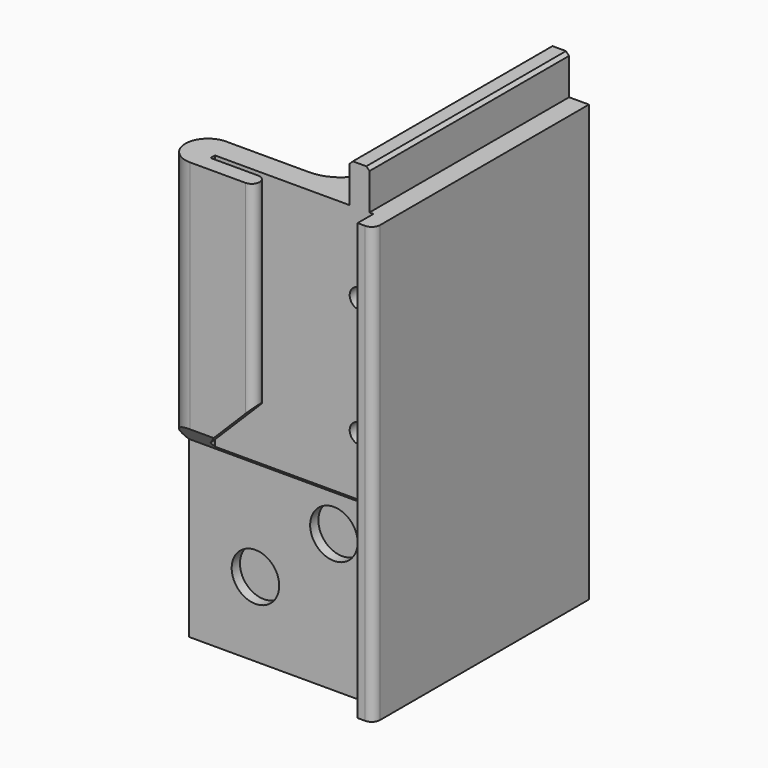
from build123d import *

# Parameters (mm, degrees)
F1_DEPTH  = 69.85
F2_W      = 3.175
F2_H      = 6.35
F3_DEPTH  = 40.005
F4_SIZE   = 0.508
F5_R      = 1.5875
F6_DEPTH  = 1.651
F7_R      = 1.5875
F8_DEPTH  = 1.651
F9_W      = 30.2895
F9_H      = 4.2418
F10_DEPTH = 27.94
F11_R     = 3.81
F12_DEPTH = 1.651
F14_DEPTH = 30.2905
F16_DEPTH = 2.54


with BuildPart() as f1:
    # F0 (on Top) → F1 (new body)
    with BuildSketch(Plane.XY):
        with BuildLine():
            Line((2.54, 40.005), (-6.985, 40.005))
            Line((-6.985, 40.005), (-6.985, 10.16))
            ThreePointArc((-6.985, 10.16), (-8.8448719395, 5.6698719395), (-13.335, 3.81))
            Line((-13.335, 3.81), (-26.67, 3.81))
            ThreePointArc((-26.67, 3.81), (-30.2895, 0.1905), (-26.67, -3.429))
            Line((-26.67, -3.429), (-17.78, -3.429))
            ThreePointArc((-17.78, -3.429), (-16.51, -2.159), (-17.78, -0.889))
            Line((-17.78, -0.889), (-25.4, -0.889))
            Line((-25.4, -0.889), (-25.4, 0))
            Line((-25.4, 0), (0, 0))
            Line((0, 0), (0, -3.175))
            Line((0, -3.175), (1.2192, -3.175))
            ThreePointArc((1.2192, -3.175), (2.1531466366, -2.7881466366), (2.54, -1.8542))
            Line((2.54, -1.8542), (2.54, 40.005))
        make_face()
    extrude(amount=F1_DEPTH)

    # F2 (on face) → F3 (join, through all)
    with BuildSketch(Plane(origin=(0, 40.005, 0), x_dir=(-1, 0, 0), z_dir=(0, 1, 0))):
        with Locations((2.2225, 73.025)):
            Rectangle(F2_W, F2_H)
    extrude(amount=-F3_DEPTH)

    # F4
    f4_edges = [f1.edges().sort_by_distance(p)[0] for p in [
        (-0.635, 20.0025, 76.2),
        (-3.81, 20.0025, 76.2),
    ]]
    chamfer(f4_edges, length=F4_SIZE)

    # F5 (on face) → F6 (cut)
    with BuildSketch(Plane(origin=(0, 40.005, 0), x_dir=(-1, 0, 0), z_dir=(0, 1, 0))):
        with Locations((2.2225, 6.35)):
            Circle(F5_R)
        with Locations((2.2225, 31.75)):
            Circle(F5_R)
        with Locations((2.2225, 57.15)):
            Circle(F5_R)
    extrude(amount=-F6_DEPTH, mode=Mode.SUBTRACT)

    # F7 (on face) → F8 (cut)
    with BuildSketch(Plane.XZ):
        with Locations((-2.2225, 57.15)):
            Circle(F7_R)
        with Locations((-2.2225, 38.1)):
            Circle(F7_R)
    extrude(amount=-F8_DEPTH, mode=Mode.SUBTRACT)

    # F9 (on face) → F10 (cut)
    with BuildSketch(Plane(origin=(0, 0, 0), x_dir=(1, 0, 0), z_dir=(0, 0, -1))):
        with Locations((-15.14475, 1.3081)):
            Rectangle(F9_W, F9_H)
    extrude(amount=-F10_DEPTH, mode=Mode.SUBTRACT)

    # F11 (on face) → F12 (cut)
    with BuildSketch(Plane.XZ.offset(-0.8128)):
        with Locations((-6.985, 22.098)):
            Circle(F11_R)
        with Locations((-19.558, 11.938)):
            Circle(F11_R)
    extrude(amount=-F12_DEPTH, mode=Mode.SUBTRACT)

    # F13 (on face) → F14 (cut, through all)
    with BuildSketch(Plane(origin=(0, 0, 0), x_dir=(0, -1, 0), z_dir=(-1, 0, 0))):
        Polygon((3.429, 32.1818), (-0.8128, 27.94), (3.429, 27.94), align=None)
    extrude(amount=F14_DEPTH, mode=Mode.SUBTRACT)

    # F15 (on face) → F16 (cut, through all)
    with BuildSketch(Plane.XZ.offset(3.429)):
        Polygon((-12.7, 42.3418), (-25.4, 29.6418), (-12.7, 29.6418), align=None)
    extrude(amount=-F16_DEPTH, mode=Mode.SUBTRACT)


solid = f1.part
